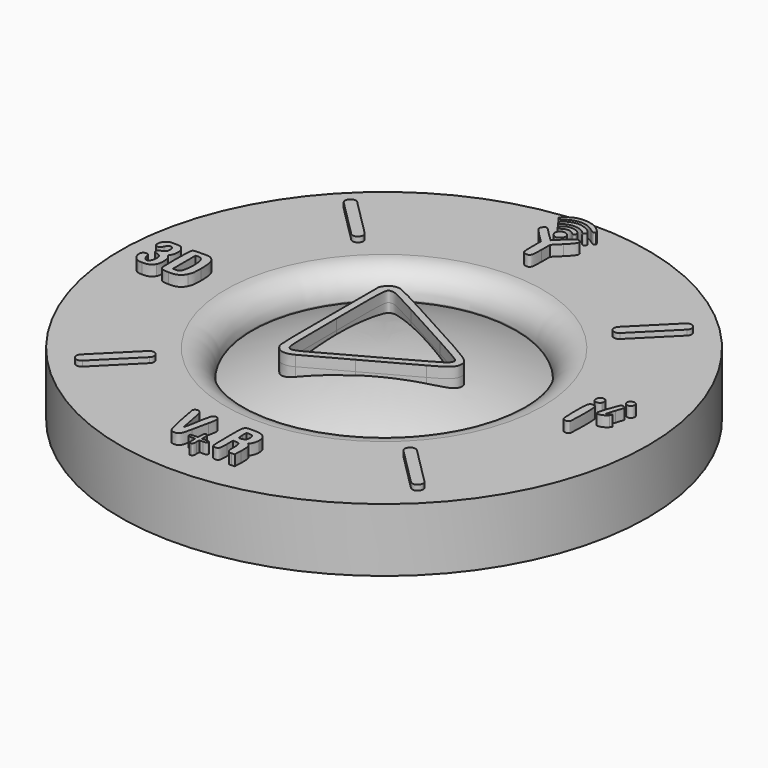
from build123d import *

# Parameters (mm, degrees)
F0_R      = 50
F0_R_2    = 25
F1_DEPTH  = 25
F4_R      = 5
F6_DEPTH  = 1
F8_DEPTH  = 2
F9_DEPTH  = 10
F10_DEPTH = 5
F11_DEPTH = 8


# Not quite as in the source:
# - ends of sketch curves that miss each other by under 0.0002 mm in the source are joined


with BuildPart() as f1:
    # F0 (on Top) → F1 (new body)
    with BuildSketch(Plane.XY):
        Circle(F0_R)
        Circle(F0_R_2, mode=Mode.SUBTRACT)
    extrude(amount=F1_DEPTH)

    # F2 (on Front) → F3 (revolve)
    with BuildSketch(Plane.XZ):
        with BuildLine():
            Line((0, 25), (0, 0))
            Line((0, 0), (50, 0))
            ThreePointArc((50, 0), (27.9508497187, 18.4016994375), (0, 25))
        make_face()
    revolve(axis=Axis((0, 0, 12.5), (0, 0, -1)))

    # F4
    f4_edges = [f1.edges().sort_by_distance(p)[0] for p in [
        (-25, 0, 25),
    ]]
    fillet(f4_edges, radius=F4_R)

    # F5 (on face) → F6 (join)
    with BuildSketch(Plane.XY.offset(25)):
        with BuildLine():
            Line((-32.5190551926, 31.1048416302), (-25.4558441227, 24.0416305603))
            ThreePointArc((-25.4558441227, 24.0416305603), (-24.0416305603, 24.0416305603), (-24.0416305603, 25.4558441227))
            Line((-24.0416305603, 25.4558441227), (-31.1048416302, 32.5190551926))
            ThreePointArc((-31.1048416302, 32.5190551926), (-31.1087808531, 32.5229725904), (-31.1126983722, 32.5269119346))
            ThreePointArc((-31.1126983722, 32.5269119346), (-32.5269119346, 32.5269119346), (-32.5269119346, 31.1126983722))
            ThreePointArc((-32.5269119346, 31.1126983722), (-32.5229725904, 31.1087808531), (-32.5190551926, 31.1048416302))
        make_face()
        with BuildLine():
            Line((25.4558441227, 24.0416305603), (32.5190551926, 31.1048416302))
            ThreePointArc((32.5190551926, 31.1048416302), (32.5229725904, 31.1087808531), (32.5269119346, 31.1126983722))
            ThreePointArc((32.5269119346, 31.1126983722), (32.5269119346, 32.5269119346), (31.1126983722, 32.5269119346))
            ThreePointArc((31.1126983722, 32.5269119346), (31.1087808531, 32.5229725904), (31.1048852801, 32.5190115427))
            Line((31.1048852801, 32.5190115427), (24.0416305603, 25.4558441227))
            ThreePointArc((24.0416305603, 25.4558441227), (24.0416305603, 24.0416305603), (25.4558441227, 24.0416305603))
        make_face()
        with BuildLine():
            Line((32.5190551926, -31.1048416302), (25.4558441227, -24.0416305603))
            ThreePointArc((25.4558441227, -24.0416305603), (24.0416305603, -24.0416305603), (24.0416305603, -25.4558441227))
            Line((24.0416305603, -25.4558441227), (31.1048416302, -32.5190551926))
            ThreePointArc((31.1048416302, -32.5190551926), (31.1087808531, -32.5229725904), (31.1126983722, -32.5269119346))
            ThreePointArc((31.1126983722, -32.5269119346), (32.5269119346, -32.5269119346), (32.5269119346, -31.1126983722))
            ThreePointArc((32.5269119346, -31.1126983722), (32.5229725904, -31.1087808531), (32.5190551926, -31.1048416302))
        make_face()
        with BuildLine():
            Line((-31.1048416302, -32.5190551926), (-24.0416305603, -25.4558441227))
            ThreePointArc((-24.0416305603, -25.4558441227), (-24.0416305603, -24.0416305603), (-25.4558441227, -24.0416305603))
            Line((-25.4558441227, -24.0416305603), (-32.5190551926, -31.1048416302))
            ThreePointArc((-32.5190551926, -31.1048416302), (-32.5229725904, -31.1087808531), (-32.5269119346, -31.1126983722))
            ThreePointArc((-32.5269119346, -31.1126983722), (-32.5269119346, -32.5269119346), (-31.1126983722, -32.5269119346))
            ThreePointArc((-31.1126983722, -32.5269119346), (-31.1087808531, -32.5229725904), (-31.1048416302, -32.5190551926))
        make_face()
    extrude(amount=F6_DEPTH)

    # F7 (on face) → F8, piece 2 (join)
    with BuildSketch(Plane.XY.offset(25)):
        with BuildLine():
            add(Edge.make_bspline(
                [(-1.161690177, -44.6288233305), (-1.2198826643, -44.5706308432), (-1.2675113585, -44.2134859056), (-1.2675113585, -43.8351803139)],
                knots=[0, 0, 0, 0, 1, 1, 1, 1], degree=3))
            add(Edge.make_bspline(
                [(-0.7249950689, -44.6382958853), (-1.0358739824, -44.7575977178), (-1.0329102784, -44.7576624757), (-1.161690177, -44.6288233305)],
                knots=[0, 0, 0, 0, 1, 1, 1, 1], degree=3))
            add(Edge.make_bspline(
                [(-0.473915188, -43.8446528687), (-0.473915188, -44.3340691164), (-0.5487669713, -44.5706735558), (-0.7249950689, -44.6382958853)],
                knots=[0, 0, 0, 0, 1, 1, 1, 1], degree=3))
            Line((-0.473915188, -43.8446528687), (-0.473915188, -43.1473502119))
            Line((-0.473915188, -43.1473502119), (0.2403650425, -43.1473502119))
            add(Edge.make_bspline(
                [(0.9546507843, -42.829889423), (0.9546507843, -43.1003167386), (0.8488309806, -43.1473502119), (0.2403650425, -43.1473502119)],
                knots=[0, 0, 0, 0, 1, 1, 1, 1], degree=3))
            add(Edge.make_bspline(
                [(0.249063259, -42.5124341453), (0.8488309806, -42.5124341453), (0.9546507843, -42.5600683508), (0.9546507843, -42.829889423)],
                knots=[0, 0, 0, 0, 1, 1, 1, 1], degree=3))
            Line((0.249063259, -42.5124341453), (-0.4565228886, -42.5124341453))
            Line((-0.4565228886, -42.5124341453), (-0.5048763194, -41.7584642548))
            add(Edge.make_bspline(
                [(-0.87071534, -41.0044984977), (-0.604601998, -41.0044984977), (-0.5454312542, -41.1264443787), (-0.5048763194, -41.7584642548)],
                knots=[0, 0, 0, 0, 1, 1, 1, 1], degree=3))
            add(Edge.make_bspline(
                [(-1.2365543607, -41.7584642548), (-1.1959994259, -41.1264443787), (-1.1368300598, -41.0044984977), (-0.87071534, -41.0044984977)],
                knots=[0, 0, 0, 0, 1, 1, 1, 1], degree=3))
            Line((-1.2365543607, -41.7584642548), (-1.2849077915, -42.5124341453))
            Line((-1.2849077915, -42.5124341453), (-1.9904898055, -42.5124341453))
            add(Edge.make_bspline(
                [(-2.6960759531, -42.829889423), (-2.6960759531, -42.5600449278), (-2.5902561494, -42.5124341453), (-1.9904898055, -42.5124341453)],
                knots=[0, 0, 0, 0, 1, 1, 1, 1], degree=3))
            add(Edge.make_bspline(
                [(-1.9817971004, -43.1473502119), (-2.5902561494, -43.1473502119), (-2.6960759531, -43.1003167386), (-2.6960759531, -42.829889423)],
                knots=[0, 0, 0, 0, 1, 1, 1, 1], degree=3))
            Line((-1.9817971004, -43.1473502119), (-1.2675113585, -43.1473502119))
            Line((-1.2675113585, -43.1473502119), (-1.2675113585, -43.8351803139))
        make_face()
        with BuildLine():
            add(Edge.make_bspline(
                [(-5.7321888921, -43.2040615361), (-6.0594474028, -42.8123593409), (-7.4597334936, -36.4631380499), (-7.2891503496, -36.1444110387)],
                knots=[0, 0, 0, 0, 1, 1, 1, 1], degree=3))
            add(Edge.make_bspline(
                [(-4.902514344, -43.4648123787), (-5.2757509132, -43.4648123787), (-5.5992879155, -43.3631301869), (-5.7321888921, -43.2040615361)],
                knots=[0, 0, 0, 0, 1, 1, 1, 1], degree=3))
            add(Edge.make_bspline(
                [(-3.4939792081, -41.0838681729), (-3.9204053779, -43.1722888652), (-4.093452075, -43.4648123787), (-4.902514344, -43.4648123787)],
                knots=[0, 0, 0, 0, 1, 1, 1, 1], degree=3))
            add(Edge.make_bspline(
                [(-2.8372259749, -37.9927909932), (-3.0112702181, -38.7762174289), (-3.306809793, -40.167204571), (-3.4939792081, -41.0838681729)],
                knots=[0, 0, 0, 0, 1, 1, 1, 1], degree=3))
            add(Edge.make_bspline(
                [(-3.0271083296, -35.7962522832), (-2.5288243928, -35.9265546797), (-2.4866257114, -36.4146936826), (-2.8372259749, -37.9927909932)],
                knots=[0, 0, 0, 0, 1, 1, 1, 1], degree=3))
            add(Edge.make_bspline(
                [(-4.4891554774, -39.2584772477), (-3.9044294837, -35.7891551007), (-3.8198764266, -35.5889362942), (-3.0271083296, -35.7962522832)],
                knots=[0, 0, 0, 0, 1, 1, 1, 1], degree=3))
            add(Edge.make_bspline(
                [(-4.964750751, -41.1632323368), (-4.9041167558, -41.3537016455), (-4.7138692771, -40.5917692976), (-4.4891554774, -39.2584772477)],
                knots=[0, 0, 0, 0, 1, 1, 1, 1], degree=3))
            add(Edge.make_bspline(
                [(-5.8231860422, -36.6679877301), (-5.4313515756, -38.8970968724), (-5.0493575434, -40.8974606957), (-4.964750751, -41.1632323368)],
                knots=[0, 0, 0, 0, 1, 1, 1, 1], degree=3))
            add(Edge.make_bspline(
                [(-7.2891503496, -36.1444110387), (-6.9142590112, -35.4439173366), (-5.9796754024, -35.7777081211), (-5.8231860422, -36.6679877301)],
                knots=[0, 0, 0, 0, 1, 1, 1, 1], degree=3))
        make_face()
        with BuildLine():
            add(Edge.make_bspline(
                [(2.2562859008, -43.2743361809), (2.1195449227, -43.1375896915), (2.065809703, -42.086867739), (2.065809703, -39.5497703625)],
                knots=[0, 0, 0, 0, 1, 1, 1, 1], degree=3))
            add(Edge.make_bspline(
                [(2.7800651326, -43.4648234014), (2.596735719, -43.4648234014), (2.3610199775, -43.3791129702), (2.2562859008, -43.2743361809)],
                knots=[0, 0, 0, 0, 1, 1, 1, 1], degree=3))
            add(Edge.make_bspline(
                [(3.4943522523, -41.6076914952), (3.4943522523, -43.1609452225), (3.3774753937, -43.4648234014), (2.7800651326, -43.4648234014)],
                knots=[0, 0, 0, 0, 1, 1, 1, 1], degree=3))
            Line((3.4943522523, -41.6076914952), (3.4943522523, -40.1315037177))
            Line((3.4943522523, -40.1315037177), (4.044325337, -40.1315037177))
            add(Edge.make_bspline(
                [(4.9229182247, -41.8367592255), (4.9229182247, -40.4473620949), (4.7601762894, -40.1315037177), (4.044325337, -40.1315037177)],
                knots=[0, 0, 0, 0, 1, 1, 1, 1], degree=3))
            add(Edge.make_bspline(
                [(5.8823013263, -43.437634758), (5.1227099051, -43.509889339), (4.9229182247, -43.176506391), (4.9229182247, -41.8367592255)],
                knots=[0, 0, 0, 0, 1, 1, 1, 1], degree=3))
            Line((5.8823013263, -43.437634758), (6.4308469831, -43.3854413257))
            Line((6.4308469831, -43.3854413257), (6.477701339, -42.0362464064))
            add(Edge.make_bspline(
                [(6.0021970019, -39.6596947103), (6.4627037014, -40.0887222158), (6.5330982171, -40.4405349663), (6.477701339, -42.0362464064)],
                knots=[0, 0, 0, 0, 1, 1, 1, 1], degree=3))
            add(Edge.make_bspline(
                [(5.8413096206, -39.3378414115), (5.7397900123, -39.3378414115), (5.8121534415, -39.4826743626), (6.0021970019, -39.6596947103)],
                knots=[0, 0, 0, 0, 1, 1, 1, 1], degree=3))
            add(Edge.make_bspline(
                [(6.5078950212, -37.7187455061), (6.5102951944, -38.4491945265), (6.1445402211, -39.3378414115), (5.8413096206, -39.3378414115)],
                knots=[0, 0, 0, 0, 1, 1, 1, 1], degree=3))
            add(Edge.make_bspline(
                [(3.8410835799, -35.6873061919), (5.7428556754, -35.6877856754), (6.5029155575, -36.2666807088), (6.5078950212, -37.7187455061)],
                knots=[0, 0, 0, 0, 1, 1, 1, 1], degree=3))
            add(Edge.make_bspline(
                [(2.065809703, -39.5497703625), (2.065809703, -35.4398251929), (1.9522437606, -35.686909378), (3.8410835799, -35.6873061919)],
                knots=[0, 0, 0, 0, 1, 1, 1, 1], degree=3))
        make_face()
        with BuildLine():
            add(Edge.make_bspline(
                [(4.7245291713, -38.6616029609), (4.9775159636, -38.4623389879), (4.9830892703, -37.3979972239), (4.7324475382, -37.1473734035)],
                knots=[0, 0, 0, 0, 1, 1, 1, 1], degree=3))
            add(Edge.make_bspline(
                [(3.5972868881, -38.9116687618), (3.7231981527, -39.0375800263), (4.4526027808, -38.8757929245), (4.7245291713, -38.6616029609)],
                knots=[0, 0, 0, 0, 1, 1, 1, 1], degree=3))
            add(Edge.make_bspline(
                [(3.4943577636, -37.8828184215), (3.4943577636, -38.3920753657), (3.5406720117, -38.8550593967), (3.5972868881, -38.9116687618)],
                knots=[0, 0, 0, 0, 1, 1, 1, 1], degree=3))
            Line((3.4943577636, -37.8828184215), (3.4943577636, -36.9568985835))
            Line((3.4943577636, -36.9568985835), (4.0181617963, -36.9568985835))
            add(Edge.make_bspline(
                [(4.7324475382, -37.1473734035), (4.6276831493, -37.0426090146), (4.3062569766, -36.9568985835), (4.0181617963, -36.9568985835)],
                knots=[0, 0, 0, 0, 1, 1, 1, 1], degree=3))
        make_face(mode=Mode.SUBTRACT)
        with BuildLine():
            add(Edge.make_bspline(
                [(37.229598485, -3.977261647), (37.1444570961, -3.7533235634), (37.0747942061, -2.4722662804), (37.0747942061, -1.1304606427)],
                knots=[0, 0, 0, 0, 1, 1, 1, 1], degree=3))
            add(Edge.make_bspline(
                [(38.4977813604, -4.0773951622), (38.2416076563, -4.556056099), (37.4251437052, -4.4915876136), (37.229598485, -3.977261647)],
                knots=[0, 0, 0, 0, 1, 1, 1, 1], degree=3))
            add(Edge.make_bspline(
                [(38.6620940176, -1.1304606427), (38.6620940176, -2.6466701362), (38.5921486732, -3.9010540828), (38.4977813604, -4.0773951622)],
                knots=[0, 0, 0, 0, 1, 1, 1, 1], degree=3))
            add(Edge.make_bspline(
                [(38.4977813604, 1.8164738768), (38.5921486732, 1.6401327975), (38.6620940176, 0.3857474731), (38.6620940176, -1.1304606427)],
                knots=[0, 0, 0, 0, 1, 1, 1, 1], degree=3))
            add(Edge.make_bspline(
                [(37.8589302223, 2.1234962549), (38.1656343226, 2.1234962549), (38.3915771432, 2.0149097763), (38.4977813604, 1.8164738768)],
                knots=[0, 0, 0, 0, 1, 1, 1, 1], degree=3))
            add(Edge.make_bspline(
                [(37.0747942061, -1.1304606427), (37.0747942061, 1.7054693133), (37.1755339648, 2.1234962549), (37.8589302223, 2.1234962549)],
                knots=[0, 0, 0, 0, 1, 1, 1, 1], degree=3))
        make_face()
        with BuildLine():
            add(Edge.make_bspline(
                [(-44.0323031302, -3.556556482), (-44.9853068967, -2.7546575311), (-45.0002811113, -1.2651819983), (-44.0553390055, -1.2651819983)],
                knots=[0, 0, 0, 0, 1, 1, 1, 1], degree=3))
            add(Edge.make_bspline(
                [(-42.6480645806, -3.9612405552), (-43.3850940986, -3.9630399961), (-43.6363985652, -3.8896872878), (-44.0323031302, -3.556556482)],
                knots=[0, 0, 0, 0, 1, 1, 1, 1], degree=3))
            add(Edge.make_bspline(
                [(-40.6675428317, -3.008994593), (-41.0356786885, -3.7203717439), (-41.5306200191, -3.9583360977), (-42.6480645806, -3.9612405552)],
                knots=[0, 0, 0, 0, 1, 1, 1, 1], degree=3))
            add(Edge.make_bspline(
                [(-40.8300904935, -0.1195209351), (-40.3567259204, -0.6268943911), (-40.266333636, -2.2337207546), (-40.6675428317, -3.008994593)],
                knots=[0, 0, 0, 0, 1, 1, 1, 1], degree=3))
            add(Edge.make_bspline(
                [(-40.8625768784, 0.6174782707), (-41.1650923872, 0.2464131555), (-41.1647741093, 0.2392140139), (-40.8300904935, -0.1195209351)],
                knots=[0, 0, 0, 0, 1, 1, 1, 1], degree=3))
            add(Edge.make_bspline(
                [(-40.5570756204, 1.8451296344), (-40.5570756204, 1.2389495099), (-40.6454562785, 0.883795531), (-40.8625768784, 0.6174782707)],
                knots=[0, 0, 0, 0, 1, 1, 1, 1], degree=3))
            add(Edge.make_bspline(
                [(-41.02024428, 3.2164276408), (-40.630283657, 2.7799832971), (-40.5570756204, 2.563237466), (-40.5570756204, 1.8451296344)],
                knots=[0, 0, 0, 0, 1, 1, 1, 1], degree=3))
            add(Edge.make_bspline(
                [(-42.5947523535, 3.7348016607), (-41.5402027999, 3.7348016607), (-41.4597460199, 3.7083460208), (-41.02024428, 3.2164276408)],
                knots=[0, 0, 0, 0, 1, 1, 1, 1], degree=3))
            add(Edge.make_bspline(
                [(-44.1132724615, 3.3522730319), (-43.7630455889, 3.6812951601), (-43.5506454215, 3.7348016607), (-42.5947523535, 3.7348016607)],
                knots=[0, 0, 0, 0, 1, 1, 1, 1], degree=3))
            add(Edge.make_bspline(
                [(-44.5238715424, 1.669580805), (-44.8100887456, 2.0144520674), (-44.5938003528, 2.900843451), (-44.1132724615, 3.3522730319)],
                knots=[0, 0, 0, 0, 1, 1, 1, 1], degree=3))
            add(Edge.make_bspline(
                [(-43.9375569152, 1.4332229965), (-44.1521423149, 1.4332229965), (-44.4159849994, 1.5395829081), (-44.5238715424, 1.669580805)],
                knots=[0, 0, 0, 0, 1, 1, 1, 1], degree=3))
            add(Edge.make_bspline(
                [(-43.2979961966, 2.0681390632), (-43.4947511482, 1.567251035), (-43.6297601988, 1.4332229965), (-43.9375569152, 1.4332229965)],
                knots=[0, 0, 0, 0, 1, 1, 1, 1], degree=3))
            add(Edge.make_bspline(
                [(-42.7075935593, 2.7030606412), (-42.9580396401, 2.7030606412), (-43.1148224773, 2.5344532999), (-43.2979961966, 2.0681390632)],
                knots=[0, 0, 0, 0, 1, 1, 1, 1], degree=3))
            add(Edge.make_bspline(
                [(-41.9856415927, 1.7383729089), (-41.9856415927, 2.4009584802), (-42.2117263295, 2.7030606412), (-42.7075935593, 2.7030606412)],
                knots=[0, 0, 0, 0, 1, 1, 1, 1], degree=3))
            add(Edge.make_bspline(
                [(-42.8586542845, 0.687345079), (-42.1361181197, 0.9203850821), (-41.9856415927, 1.1015499308), (-41.9856415927, 1.7383729089)],
                knots=[0, 0, 0, 0, 1, 1, 1, 1], degree=3))
            add(Edge.make_bspline(
                [(-43.3348434012, 0.1566656938), (-43.3348434012, 0.4357071785), (-43.2110236767, 0.573689578), (-42.8586542845, 0.687345079)],
                knots=[0, 0, 0, 0, 1, 1, 1, 1], degree=3))
            add(Edge.make_bspline(
                [(-42.7870445262, -0.332457077), (-43.2264594631, -0.2425897444), (-43.3348434012, -0.1458153693), (-43.3348434012, 0.1566656938)],
                knots=[0, 0, 0, 0, 1, 1, 1, 1], degree=3))
            add(Edge.make_bspline(
                [(-41.8269118872, -1.5232805256), (-41.8269118872, -0.8363749449), (-42.1238458222, -0.4680999276), (-42.7870445262, -0.332457077)],
                knots=[0, 0, 0, 0, 1, 1, 1, 1], degree=3))
            add(Edge.make_bspline(
                [(-43.3963412935, -1.9846621447), (-43.0115158285, -3.5129413953), (-41.8269118872, -3.1646930811), (-41.8269118872, -1.5232805256)],
                knots=[0, 0, 0, 0, 1, 1, 1, 1], degree=3))
            add(Edge.make_bspline(
                [(-44.0553390055, -1.2651819983), (-43.6209751793, -1.2651819983), (-43.5610273415, -1.3306273624), (-43.3963412935, -1.9846621447)],
                knots=[0, 0, 0, 0, 1, 1, 1, 1], degree=3))
        make_face()
        with BuildLine():
            add(Edge.make_bspline(
                [(-39.1285110258, -3.6461248263), (-39.42538847, -3.3492473821), (-39.4459663035, -3.1170230521), (-39.4459663035, -0.0642742401)],
                knots=[0, 0, 0, 0, 1, 1, 1, 1], degree=3))
            add(Edge.make_bspline(
                [(-37.6602595269, -3.9633334731), (-38.5996186811, -3.9634960566), (-38.8693805067, -3.9052608567), (-39.1285110258, -3.6461248263)],
                knots=[0, 0, 0, 0, 1, 1, 1, 1], degree=3))
            add(Edge.make_bspline(
                [(-35.0114204499, -2.6271741669), (-35.5216074268, -3.6567368433), (-36.1287644301, -3.963009684), (-37.6602595269, -3.9633334731)],
                knots=[0, 0, 0, 0, 1, 1, 1, 1], degree=3))
            add(Edge.make_bspline(
                [(-34.6268829506, -0.0875030111), (-34.6244827775, -1.6350883617), (-34.6709775208, -1.9401060028), (-35.0114204499, -2.6271741669)],
                knots=[0, 0, 0, 0, 1, 1, 1, 1], degree=3))
            add(Edge.make_bspline(
                [(-35.4929073082, 3.4057561095), (-34.8371309536, 2.8539601607), (-34.6297557181, 2.0174639953), (-34.6268829506, -0.0875030111)],
                knots=[0, 0, 0, 0, 1, 1, 1, 1], degree=3))
            add(Edge.make_bspline(
                [(-37.5478041125, 3.8141658246), (-36.093339142, 3.8141658246), (-35.9426876311, 3.7842297959), (-35.4929073082, 3.4057561095)],
                knots=[0, 0, 0, 0, 1, 1, 1, 1], degree=3))
            add(Edge.make_bspline(
                [(-39.2816522685, 3.5071434465), (-39.1362075627, 3.7789086313), (-38.9371047953, 3.8141658246), (-37.5478041125, 3.8141658246)],
                knots=[0, 0, 0, 0, 1, 1, 1, 1], degree=3))
            add(Edge.make_bspline(
                [(-39.4459663035, -0.0642742401), (-39.4459663035, 1.8824094764), (-39.3796446419, 3.3240537746), (-39.2816522685, 3.5071434465)],
                knots=[0, 0, 0, 0, 1, 1, 1, 1], degree=3))
        make_face()
        with BuildLine():
            add(Edge.make_bspline(
                [(-36.5174367856, -2.3313576489), (-36.2151720412, -1.8700421654), (-36.0371031678, 0.0102482427), (-36.1841916203, 1.1875069928)],
                knots=[0, 0, 0, 0, 1, 1, 1, 1], degree=3))
            add(Edge.make_bspline(
                [(-37.3067796068, -2.6937479707), (-36.9072306917, -2.6937479707), (-36.6893385092, -2.5937109033), (-36.5174367856, -2.3313576489)],
                knots=[0, 0, 0, 0, 1, 1, 1, 1], degree=3))
            Line((-37.3067796068, -2.6937479707), (-37.8586720033, -2.6937479707))
            Line((-37.8586720033, -2.6937479707), (-37.8586720033, 0.0046570242))
            Line((-37.8586720033, 0.0046570242), (-37.8586720033, 2.7030606412))
            Line((-37.8586720033, 2.7030606412), (-37.3824828866, 2.7030606412))
            add(Edge.make_bspline(
                [(-36.1841916203, 1.1875069928), (-36.3156169451, 2.2393987198), (-36.6822179036, 2.7030606412), (-37.3824828866, 2.7030606412)],
                knots=[0, 0, 0, 0, 1, 1, 1, 1], degree=3))
        make_face(mode=Mode.SUBTRACT)
        with BuildLine():
            add(Edge.make_bspline(
                [(39.9319261509, 0.5755816039), (39.9319261509, 1.1043471886), (41.0263899501, 4.2930199277), (41.2801689924, 4.5036413216)],
                knots=[0, 0, 0, 0, 1, 1, 1, 1], degree=3))
            add(Edge.make_bspline(
                [(40.3366336471, 0.2187411658), (40.0228571653, 0.2187411658), (39.9319261509, 0.2989154915), (39.9319261509, 0.5755816039)],
                knots=[0, 0, 0, 0, 1, 1, 1, 1], degree=3))
            add(Edge.make_bspline(
                [(41.902223052, 0.9971109796), (41.4969630474, 0.5493050815), (40.8320751286, 0.2187411658), (40.3366336471, 0.2187411658)],
                knots=[0, 0, 0, 0, 1, 1, 1, 1], degree=3))
            add(Edge.make_bspline(
                [(41.5979659709, 1.1705310675), (42.0747186186, 1.6184155017), (42.331856801, 1.4718533789), (41.902223052, 0.9971109796)],
                knots=[0, 0, 0, 0, 1, 1, 1, 1], degree=3))
            add(Edge.make_bspline(
                [(41.6779529122, 2.7047487488), (41.0736810769, 0.9607914824), (41.0581791549, 0.6634276655), (41.5979659709, 1.1705310675)],
                knots=[0, 0, 0, 0, 1, 1, 1, 1], degree=3))
            add(Edge.make_bspline(
                [(42.154142029, 4.2067997009), (42.154142029, 4.1365429679), (41.9398556175, 3.460615906), (41.6779529122, 2.7047487488)],
                knots=[0, 0, 0, 0, 1, 1, 1, 1], degree=3))
            add(Edge.make_bspline(
                [(41.2801689924, 4.5036413216), (41.5086428797, 4.6932591338), (42.154142029, 4.4740042812), (42.154142029, 4.2067997009)],
                knots=[0, 0, 0, 0, 1, 1, 1, 1], degree=3))
        make_face()
        with BuildLine():
            add(Edge.make_bspline(
                [(37.272426833, 3.2591915016), (37.0042081726, 3.527417051), (37.0125467765, 4.2133870877), (37.3033232065, 4.4964724922)],
                knots=[0, 0, 0, 0, 1, 1, 1, 1], degree=3))
            add(Edge.make_bspline(
                [(38.5025927293, 3.4303188868), (38.2810107284, 2.9834609331), (37.5999609089, 2.9316932491), (37.272426833, 3.2591915016)],
                knots=[0, 0, 0, 0, 1, 1, 1, 1], degree=3))
            add(Edge.make_bspline(
                [(38.4681567205, 4.3350091795), (38.56721002, 4.1085923867), (38.6602160405, 3.748230225), (38.5025927293, 3.4303188868)],
                knots=[0, 0, 0, 0, 1, 1, 1, 1], degree=3))
            add(Edge.make_bspline(
                [(37.3033232065, 4.4964724922), (37.6303350863, 4.767865664), (38.2214142363, 4.7090131979), (38.4681567205, 4.3350091795)],
                knots=[0, 0, 0, 0, 1, 1, 1, 1], degree=3))
        make_face()
        with BuildLine():
            add(Edge.make_bspline(
                [(41.450960188, 5.4891342287), (41.2425295377, 5.7867074751), (41.2379827114, 5.8873990099), (41.4204840515, 6.1637358219)],
                knots=[0, 0, 0, 0, 1, 1, 1, 1], degree=3))
            add(Edge.make_bspline(
                [(42.7890760074, 5.8659517681), (42.7890760074, 5.121393808), (41.8865709469, 4.8672427526), (41.450960188, 5.4891342287)],
                knots=[0, 0, 0, 0, 1, 1, 1, 1], degree=3))
            add(Edge.make_bspline(
                [(41.4204840515, 6.1637358219), (41.8425838472, 6.8029231496), (42.7890760074, 6.596975342), (42.7890760074, 5.8659517681)],
                knots=[0, 0, 0, 0, 1, 1, 1, 1], degree=3))
        make_face()
        with BuildLine():
            add(Edge.make_bspline(
                [(-0.5624938931, 33.8527360139), (-0.7630626674, 34.0533020326), (-0.8119258939, 34.4970584996), (-0.8119258939, 36.1179414456)],
                knots=[0, 0, 0, 0, 1, 1, 1, 1], degree=3))
            add(Edge.make_bspline(
                [(0.0610867979, 33.6032998796), (-0.1446956706, 33.6032998796), (-0.4253064993, 33.7155458644), (-0.5624938931, 33.8527360139)],
                knots=[0, 0, 0, 0, 1, 1, 1, 1], degree=3))
            add(Edge.make_bspline(
                [(0.9340994896, 36.1179414456), (0.9340994896, 33.9341517609), (0.8192383908, 33.6032998796), (0.0610867979, 33.6032998796)],
                knots=[0, 0, 0, 0, 1, 1, 1, 1], degree=3))
            Line((0.9340994896, 36.1179414456), (0.9340994896, 38.1337121208))
            Line((0.9340994896, 38.1337121208), (2.362665462, 39.5556603942))
            add(Edge.make_bspline(
                [(3.6007552366, 41.8254925661), (4.0183013169, 41.4079464858), (3.7744701793, 40.9609259486), (2.362665462, 39.5556603942)],
                knots=[0, 0, 0, 0, 1, 1, 1, 1], degree=3))
            add(Edge.make_bspline(
                [(1.4134286722, 40.6699207995), (2.7372426561, 42.0006514707), (3.1876471343, 42.2385992905), (3.6007552366, 41.8254925661)],
                knots=[0, 0, 0, 0, 1, 1, 1, 1], degree=3))
            Line((1.4134286722, 40.6699207995), (0.0743773089, 39.323881102))
            Line((0.0743773089, 39.323881102), (-1.3791355837, 40.7492904747))
            add(Edge.make_bspline(
                [(-2.9605782562, 42.1746957139), (-2.5359088147, 42.0329697608), (-2.1785682258, 41.5332639073), (-1.3791355837, 40.7492904747)],
                knots=[0, 0, 0, 0, 1, 1, 1, 1], degree=3))
            add(Edge.make_bspline(
                [(-3.6690578386, 41.3134579243), (-3.6690578386, 41.6362054322), (-3.2124255862, 42.2587444866), (-2.9605782562, 42.1746957139)],
                knots=[0, 0, 0, 0, 1, 1, 1, 1], degree=3))
            add(Edge.make_bspline(
                [(-2.2404918663, 39.5556603942), (-3.1412856666, 40.4522807592), (-3.6690578386, 41.1016860456), (-3.6690578386, 41.3134579243)],
                knots=[0, 0, 0, 0, 1, 1, 1, 1], degree=3))
            Line((-2.2404918663, 39.5556603942), (-0.8119258939, 38.1337121208))
            Line((-0.8119258939, 38.1337121208), (-0.8119258939, 36.1179414456))
        make_face()
        with BuildLine():
            add(Edge.make_bspline(
                [(-0.6255280615, 40.9547711992), (-1.0560436193, 41.41303342), (-1.0662271323, 41.9203999867), (-0.6531961883, 42.3334295529)],
                knots=[0, 0, 0, 0, 1, 1, 1, 1], degree=3))
            add(Edge.make_bspline(
                [(0.082571241, 40.5874014137), (-0.1170633672, 40.5874014137), (-0.4357077089, 40.7527226396), (-0.6255280615, 40.9547711992)],
                knots=[0, 0, 0, 0, 1, 1, 1, 1], degree=3))
            add(Edge.make_bspline(
                [(1.0928278174, 41.6490729506), (1.0928278174, 41.1677486758), (0.5405868308, 40.5874014137), (0.082571241, 40.5874014137)],
                knots=[0, 0, 0, 0, 1, 1, 1, 1], degree=3))
            add(Edge.make_bspline(
                [(-0.6531961883, 42.3334295529), (-0.0360306559, 42.9505937075), (1.0928278174, 42.5081379083), (1.0928278174, 41.6490729506)],
                knots=[0, 0, 0, 0, 1, 1, 1, 1], degree=3))
        make_face()
        with BuildLine():
            add(Edge.make_bspline(
                [(1.0928278174, 43.124865292), (0.4415486874, 43.6299281335), (-0.0942203876, 43.6701041661), (-0.810395129, 43.2675929247)],
                knots=[0, 0, 0, 0, 1, 1, 1, 1], degree=3))
            add(Edge.make_bspline(
                [(1.8071108036, 43.2819002714), (1.8071108036, 42.7984114318), (1.5785859367, 42.7481676235), (1.0928278174, 43.124865292)],
                knots=[0, 0, 0, 0, 1, 1, 1, 1], degree=3))
            add(Edge.make_bspline(
                [(-1.0950333436, 44.0873815703), (-0.0985316056, 44.7129683761), (1.8071108036, 44.1840650088), (1.8071108036, 43.2819002714)],
                knots=[0, 0, 0, 0, 1, 1, 1, 1], degree=3))
            add(Edge.make_bspline(
                [(-1.6282630849, 43.0862723816), (-1.8868851862, 43.344893105), (-1.6905339376, 43.7135332462), (-1.0950333436, 44.0873815703)],
                knots=[0, 0, 0, 0, 1, 1, 1, 1], degree=3))
            add(Edge.make_bspline(
                [(-0.810395129, 43.2675929247), (-1.2834262682, 43.0017303471), (-1.4964877923, 42.9544984668), (-1.6282630849, 43.0862723816)],
                knots=[0, 0, 0, 0, 1, 1, 1, 1], degree=3))
        make_face()
        with BuildLine():
            add(Edge.make_bspline(
                [(2.0365202348, 44.328009262), (1.366100344, 45.1358177092), (-0.6587419386, 45.2807650198), (-1.595729854, 44.5880160785)],
                knots=[0, 0, 0, 0, 1, 1, 1, 1], degree=3))
            add(Edge.make_bspline(
                [(2.8388532009, 44.4654708432), (2.8388532009, 44.0129968701), (2.3652902208, 43.9318690887), (2.0365202348, 44.328009262)],
                knots=[0, 0, 0, 0, 1, 1, 1, 1], degree=3))
            add(Edge.make_bspline(
                [(0.0694061122, 45.9842045143), (1.252183056, 45.9842045143), (2.8388532009, 45.1140949022), (2.8388532009, 44.4654708432)],
                knots=[0, 0, 0, 0, 1, 1, 1, 1], degree=3))
            add(Edge.make_bspline(
                [(-2.618804347, 44.4852729606), (-2.8299134914, 45.0354141401), (-1.1283326459, 45.9842045143), (0.0694061122, 45.9842045143)],
                knots=[0, 0, 0, 0, 1, 1, 1, 1], degree=3))
            add(Edge.make_bspline(
                [(-1.595729854, 44.5880160785), (-2.1524170855, 44.1764401189), (-2.4873845335, 44.1428018714), (-2.618804347, 44.4852729606)],
                knots=[0, 0, 0, 0, 1, 1, 1, 1], degree=3))
        make_face()
        with BuildLine():
            add(Edge.make_bspline(
                [(2.5570670865, 45.7519980959), (1.1002556782, 46.9047205181), (-0.9782088424, 46.9012704414), (-2.4959766573, 45.7435988677)],
                knots=[0, 0, 0, 0, 1, 1, 1, 1], degree=3))
            add(Edge.make_bspline(
                [(3.7447918041, 45.4572259701), (3.5981580343, 45.0751051779), (3.1783881426, 45.2703624324), (2.5570670865, 45.7519980959)],
                knots=[0, 0, 0, 0, 1, 1, 1, 1], degree=3))
            add(Edge.make_bspline(
                [(1.6784121967, 47.1953219642), (2.6919852007, 46.8534378289), (3.8929356714, 45.8432832116), (3.7447918041, 45.4572259701)],
                knots=[0, 0, 0, 0, 1, 1, 1, 1], degree=3))
            add(Edge.make_bspline(
                [(-1.4004863777, 47.2754425546), (-0.4423791431, 47.546204682), (0.7284809825, 47.5157409459), (1.6784121967, 47.1953219642)],
                knots=[0, 0, 0, 0, 1, 1, 1, 1], degree=3))
            add(Edge.make_bspline(
                [(-3.4777122325, 45.7982530975), (-3.4052509776, 46.1745181286), (-2.1582797357, 47.0612815253), (-1.4004863777, 47.2754425546)],
                knots=[0, 0, 0, 0, 1, 1, 1, 1], degree=3))
            add(Edge.make_bspline(
                [(-2.4959766573, 45.7435988677), (-3.0389503852, 45.3294546402), (-3.5623824049, 45.3585873963), (-3.4777122325, 45.7982530975)],
                knots=[0, 0, 0, 0, 1, 1, 1, 1], degree=3))
        make_face()
    extrude(amount=F8_DEPTH)



with BuildPart() as f8:
    # F7 (on face) → F8 (new body)
    with BuildSketch(Plane.XY.offset(25)):
        with BuildLine():
            add(Edge.make_bspline(
                [(-9.286972665, -13.0609817694), (-9.5558637045, -12.8970108131), (-9.9130031309, -12.4865674266), (-10.0806225708, -12.1488773942)],
                knots=[0, 0, 0, 0, 1, 1, 1, 1], degree=3))
            add(Edge.make_bspline(
                [(-6.4865988906, -12.8916772481), (-7.5767252931, -13.4456336282), (-8.5588163474, -13.5050082904), (-9.286972665, -13.0609817694)],
                knots=[0, 0, 0, 0, 1, 1, 1, 1], degree=3))
            add(Edge.make_bspline(
                [(1.4695093883, -8.5528269317), (-2.3991577555, -10.6814539688), (-5.979412819, -12.6339383335), (-6.4865988906, -12.8916772481)],
                knots=[0, 0, 0, 0, 1, 1, 1, 1], degree=3))
            add(Edge.make_bspline(
                [(10.7922544878, -3.4374241542), (9.5334063845, -4.1222657513), (5.3381765322, -6.4241930055), (1.4695093883, -8.5528269317)],
                knots=[0, 0, 0, 0, 1, 1, 1, 1], degree=3))
            add(Edge.make_bspline(
                [(14.6145302253, 0.2093468443), (14.6145302253, -1.0782206672), (13.93217836, -1.7292407658), (10.7922544878, -3.4374241542)],
                knots=[0, 0, 0, 0, 1, 1, 1, 1], degree=3))
            add(Edge.make_bspline(
                [(9.8526431914, 3.9939087245), (13.8256379532, 1.8146383096), (14.6145302253, 1.1876585215), (14.6145302253, 0.2093468443)],
                knots=[0, 0, 0, 0, 1, 1, 1, 1], degree=3))
            add(Edge.make_bspline(
                [(-0.2393036666, 9.541124972), (3.3469793863, 7.5676053356), (7.8883591236, 5.0713577486), (9.8526431914, 3.9939087245)],
                knots=[0, 0, 0, 0, 1, 1, 1, 1], degree=3))
            add(Edge.make_bspline(
                [(-7.4767529835, 13.3098666524), (-7.0824549638, 13.2105805002), (-3.8256115204, 11.5146459863), (-0.2393036666, 9.541124972)],
                knots=[0, 0, 0, 0, 1, 1, 1, 1], degree=3))
            add(Edge.make_bspline(
                [(-9.9510504221, 12.4778263767), (-9.5240138753, 13.1230981847), (-8.5728963528, 13.5858755417), (-7.4767529835, 13.3098666524)],
                knots=[0, 0, 0, 0, 1, 1, 1, 1], degree=3))
            Line((-9.9510504221, 12.4778263767), (-10.3853825583, 11.8215236926))
            Line((-10.3853825583, 11.8215236926), (-10.3853825583, 0.1433103928))
            add(Edge.make_bspline(
                [(-10.0806225708, -12.1488773942), (-10.3728085169, -11.5602094399), (-10.3853825583, -11.0536227228), (-10.3853825583, 0.1433103928)],
                knots=[0, 0, 0, 0, 1, 1, 1, 1], degree=3))
        make_face()
        with BuildLine():
            add(Edge.make_bspline(
                [(-4.7671007938, -10.4819378536), (-3.3174830158, -9.6845512834), (-1.7743025754, -8.8355816579), (-1.337792096, -8.5953370018)],
                knots=[0, 0, 0, 0, 1, 1, 1, 1], degree=3))
            add(Edge.make_bspline(
                [(-8.6753694168, -11.5022980292), (-8.2031994189, -12.2227509208), (-7.6866730639, -12.0879003202), (-4.7671007938, -10.4819378536)],
                knots=[0, 0, 0, 0, 1, 1, 1, 1], degree=3))
            add(Edge.make_bspline(
                [(-8.999651823, -0.0720259222), (-8.9598161135, -10.2936827115), (-8.9368753081, -11.1032892219), (-8.6753694168, -11.5022980292)],
                knots=[0, 0, 0, 0, 1, 1, 1, 1], degree=3))
            add(Edge.make_bspline(
                [(-7.8979599479, 11.8777045537), (-9.0981167908, 11.8777045537), (-9.0483235317, 12.4177448898), (-8.999651823, -0.0720259222)],
                knots=[0, 0, 0, 0, 1, 1, 1, 1], degree=3))
            add(Edge.make_bspline(
                [(-2.2274420385, 9.1172588032), (-6.436698161, 11.4334355354), (-7.3493123319, 11.8777045537), (-7.8979599479, 11.8777045537)],
                knots=[0, 0, 0, 0, 1, 1, 1, 1], degree=3))
            add(Edge.make_bspline(
                [(7.630421802, 3.7044798085), (4.96773695, 5.1632642639), (0.5316920216, 7.5990142604), (-2.2274420385, 9.1172588032)],
                knots=[0, 0, 0, 0, 1, 1, 1, 1], degree=3))
            add(Edge.make_bspline(
                [(12.8288234487, 0.7229935427), (12.6323977976, 0.9040274979), (10.2931190544, 2.245695353), (7.630421802, 3.7044798085)],
                knots=[0, 0, 0, 0, 1, 1, 1, 1], degree=3))
            add(Edge.make_bspline(
                [(12.7494606627, -0.6509870913), (13.2793905104, -0.0800862052), (13.300657257, 0.2881350769), (12.8288234487, 0.7229935427)],
                knots=[0, 0, 0, 0, 1, 1, 1, 1], degree=3))
            add(Edge.make_bspline(
                [(5.8844005519, -4.6398847225), (9.4908604909, -2.6659048921), (12.5045782438, -0.914803597), (12.7494606627, -0.6509870913)],
                knots=[0, 0, 0, 0, 1, 1, 1, 1], degree=3))
            add(Edge.make_bspline(
                [(-1.337792096, -8.5953370018), (-0.9012885058, -8.3550923457), (2.3486961191, -6.5751393712), (5.8844005519, -4.6398847225)],
                knots=[0, 0, 0, 0, 1, 1, 1, 1], degree=3))
        make_face(mode=Mode.SUBTRACT)
    extrude(amount=F8_DEPTH)


with BuildPart() as f1_1:
    add(f1.part)
    # F9 (add): a face of the model
    f9_faces = [f8.part.faces().sort_by_distance(p)[0] for p in [
        (-8.7372801562, 12.9309578521, 27),
    ]]

    add(f8.part)  # F9 merges F8
    extrude(f9_faces, amount=-F9_DEPTH)

    # F10 (cut): a face of the model
    f10_faces = [f1_1.faces().sort_by_distance(p)[0] for p in [
        (0, 0, 0),
    ]]
    extrude(f10_faces, amount=-F10_DEPTH, mode=Mode.SUBTRACT)

    # F11 (cut): a face of the model
    f11_faces = [f1_1.faces().sort_by_distance(p)[0] for p in [
        (0, 0, 5),
    ]]
    extrude(f11_faces, amount=-F11_DEPTH, mode=Mode.SUBTRACT)


solid = f1_1.part
